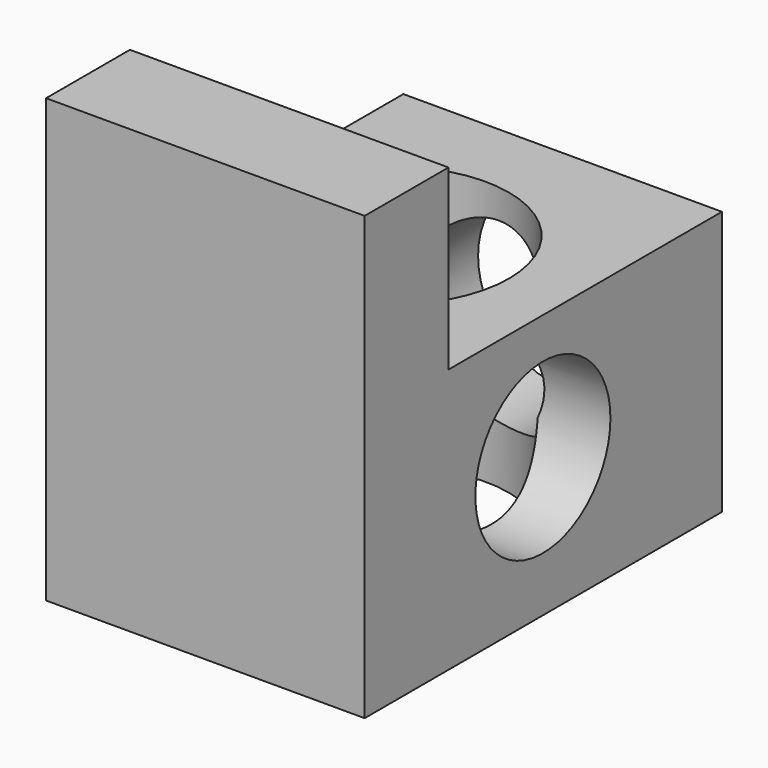
from build123d import *

# Parameters (mm, degrees)
F0_W      = 45.4768538475
F0_H      = 37.7318039536
F1_DEPTH  = 63.754
F2_R      = 16.6615499076
F3_DEPTH  = 75.184
F4_W      = 45.4768538475
F4_H      = 14.9607213655
F5_DEPTH  = 25.4
F8_R      = 12.0524100186
F10_DEPTH = 59.436
F11_R     = 12.7
F12_DEPTH = 25.4


# Not quite as in the source:
# - the program builds the solid bodies; features that only make, move or delete a surface that nothing else refers to are left out


with BuildPart() as f1:
    # F0 (on Front) → F1 (new body)
    with BuildSketch(Plane.XZ):
        with Locations((22.7384269238, 18.8659019768)):
            Rectangle(F0_W, F0_H)
    extrude(amount=F1_DEPTH)

    # F2 (on face) → F3 (cut)
    with BuildSketch(Plane.XY.offset(37.7318039536)):
        with Locations((20.3596297652, -27.4416878819)):
            Circle(F2_R)
    extrude(amount=-F3_DEPTH, mode=Mode.SUBTRACT)

    # F4 (on face) → F5 (join)
    with BuildSketch(Plane.XY.offset(37.7318039536)):
        with Locations((22.7384269238, -56.2736393173)):
            Rectangle(F4_W, F4_H)
    extrude(amount=F5_DEPTH)

    # F8 (on face) → F10 (cut)
    with BuildSketch(Plane.YZ.offset(45.4768538475)):
        with Locations((-31.9488979876, 19.8562797159)):
            Circle(F8_R)
    extrude(amount=-F10_DEPTH, mode=Mode.SUBTRACT)

    # F11 (on face) → F12 (cut)
    with BuildSketch(Plane(origin=(0, 0, 0), x_dir=(-1, 0, 0), z_dir=(0, 1, 0))):
        with Locations((-23.3701635152, 20.8852831274)):
            Circle(F11_R)
    extrude(amount=-F12_DEPTH, mode=Mode.SUBTRACT)


solid = f1.part
